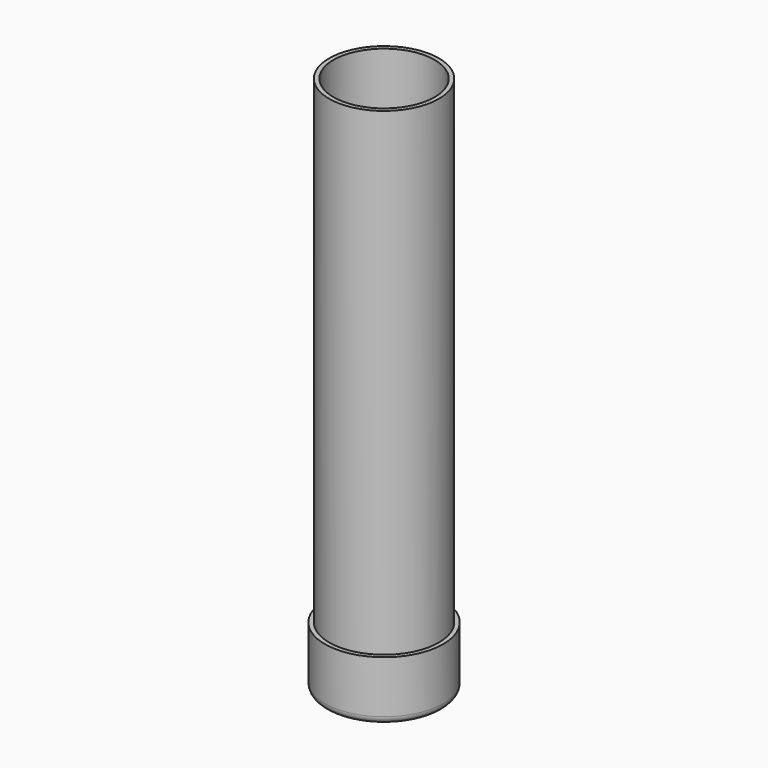
from build123d import *

# Parameters (mm, degrees)
F0_R     = 55
F0_R_2   = 51
F0_R_3   = 47
F1_DEPTH = 5
F2_DEPTH = 500
F3_DEPTH = 50
F4_R     = 10
F5_DEPTH = 25
F6_DEPTH = 25
F7_DEPTH = 25


# Not quite as in the source:
# - a fillet or chamfer that OpenCascade refuses, or shapes differently, is made with other operations: its cross-section is extruded or revolved along the edge and cut away or added


with BuildPart() as f1:
    # F0 (on Top) → F1 (new body)
    with BuildSketch(Plane.XY):
        Circle(F0_R)
        Circle(F0_R_2, mode=Mode.SUBTRACT)
        Circle(F0_R_2)
        Circle(F0_R_3, mode=Mode.SUBTRACT)
        Circle(F0_R_3)
    extrude(amount=F1_DEPTH)

    # F0 (on Top) → F2 (join)
    with BuildSketch(Plane.XY):
        Circle(F0_R_2)
        Circle(F0_R_3, mode=Mode.SUBTRACT)
    extrude(amount=F2_DEPTH)

    # F3 (add): a face of the model
    f3_faces = [f1.faces().sort_by_distance(p)[0] for p in [
        (-53.4443650814, 0, 5),
    ]]
    extrude(f3_faces, amount=F3_DEPTH)

    # F4
    f4_edges = [f1.edges().sort_by_distance(p)[0] for p in [
        (-55, 0, 0),
    ]]
    fillet(f4_edges, radius=F4_R)

    # F0 (on Top) → F5 (join)
    with BuildSketch(Plane.XY):
        Circle(F0_R)
        Circle(F0_R_2, mode=Mode.SUBTRACT)
    extrude(amount=F5_DEPTH)

    # F0 (on Top) → F6 (join)
    with BuildSketch(Plane.XY):
        Circle(F0_R)
        Circle(F0_R_2, mode=Mode.SUBTRACT)
    extrude(amount=F6_DEPTH)

    # F0 (on Top) → F7 (join)
    with BuildSketch(Plane.XY):
        Circle(F0_R)
        Circle(F0_R_2, mode=Mode.SUBTRACT)
    extrude(amount=F7_DEPTH)

    # F8: fillet of radius 7 on 1 edges, made by hand

    # F8_s1 → F8_t2 (revolve, cut)
    with BuildSketch(Plane.XZ):
        with BuildLine():
            ThreePointArc((55, 6.3245553203), (53.9160797831, 2.5828979336), (51, 0))
            Line((51, 0), (55, 0))
            Line((55, 0), (55, 6.3245553203))
        make_face()
    revolve(axis=Axis((0, 0, 0), (0, 0, 1)), mode=Mode.SUBTRACT)


solid = f1.part
